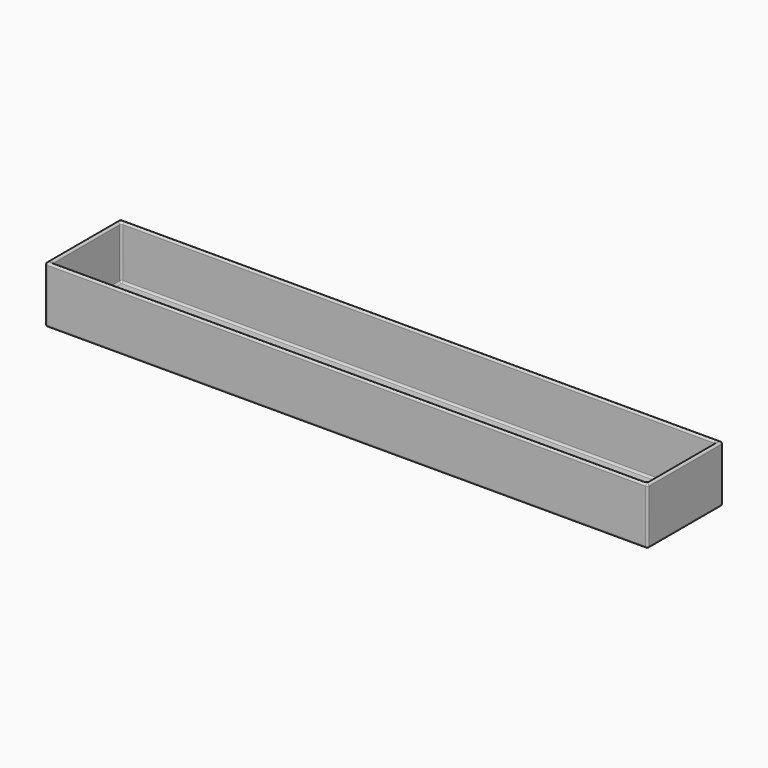
from build123d import *

# Parameters (mm, degrees)
F0_W     = 160
F0_H     = 25
F1_DEPTH = 15
F2_T     = -1
F3_R     = 0.5
F4_R     = 0.5
F5_R     = 0.49999


# Not quite as in the source:
# - a fillet or chamfer is up to 0.001 mm smaller than in the source, because OpenCascade refuses the exact size


with BuildPart() as f1:
    # F0 (on Top) → F1 (new body)
    with BuildSketch(Plane.XY):
        with Locations((30.8671402, -38.0363363773)):
            Rectangle(F0_W, F0_H)
    extrude(amount=F1_DEPTH)

    # F2
    f2_openings = [f1.faces().sort_by_distance(p)[0] for p in [
        (30.86714, -38.036336, 15),
    ]]
    offset(amount=F2_T, openings=f2_openings)

    # F3
    f3_edges = [f1.edges().sort_by_distance(p)[0] for p in [
        (30.86714, -25.536336, 0),
        (110.86714, -38.036336, 0),
        (-49.13286, -38.036336, 0),
        (30.86714, -50.536336, 0),
        (110.86714, -25.536336, 7.5),
        (-49.13286, -25.536336, 7.5),
        (-49.13286, -50.536336, 7.5),
        (110.86714, -50.536336, 7.5),
    ]]
    fillet(f3_edges, radius=F3_R)

    # F4
    f4_edges = [f1.edges().sort_by_distance(p)[0] for p in [
        (-48.13286, -38.036336, 1),
        (30.86714, -26.536336, 1),
        (30.86714, -49.536336, 1),
        (109.86714, -38.036336, 1),
        (-48.13286, -26.536336, 8),
        (-48.13286, -49.536336, 8),
        (109.86714, -26.536336, 8),
        (109.86714, -49.536336, 8),
    ]]
    fillet(f4_edges, radius=F4_R)

    # F5 (radius 0.5 in the source; OpenCascade refuses exactly that, so slightly less here)
    f5_edges = [f1.edges().sort_by_distance(p)[0] for p in [
        (30.86714, -25.536336, 15),
        (30.86714, -26.536336, 15),
        (30.86714, -49.536336, 15),
        (30.86714, -50.536336, 15),
        (109.86714, -38.036336, 15),
        (110.86714, -38.036336, 15),
        (-49.13286, -38.036336, 15),
        (-48.13286, -38.036336, 15),
        (-47.986413, -49.38989, 15),
        (-47.986413, -26.682783, 15),
        (-48.986413, -25.682783, 15),
        (-48.986413, -50.38989, 15),
        (109.720694, -26.682783, 15),
        (110.720694, -25.682783, 15),
        (109.720694, -49.38989, 15),
        (110.720694, -50.38989, 15),
    ]]
    fillet(f5_edges, radius=F5_R)


solid = f1.part
